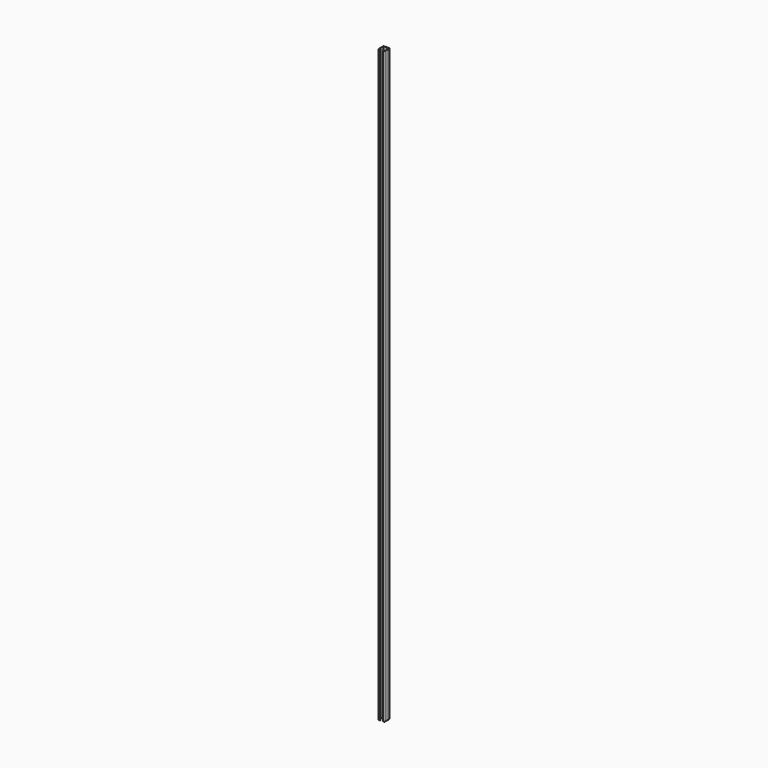
from build123d import *

# Parameters (mm, degrees)
F1_DEPTH    = 450
F2_T1_DEPTH = 452.5
F2_T3_DEPTH = 7.2
F3_R        = 0.5
F4_DEPTH    = 25


# Not quite as in the source:
# - a fillet or chamfer that OpenCascade refuses, or shapes differently, is made with other operations: its cross-section is extruded or revolved along the edge and cut away or added


with BuildPart() as f1:
    # F0 (on Top) → F1 (new body)
    with BuildSketch(Plane.XY):
        Polygon((-3.0933290763, 0), (-1.5933290763, 0), (-1.5933290763, 0.3), (-2.7933290763, 0.3), (-2.7933290763, 4.4), (1.6066709237, 4.4), (1.6066709237, 0.3), (0.4066709237, 0.3), (0.4066709237, 0), (1.9066709237, 0), (1.9066709237, 4.7), (-3.0933290763, 4.7), align=None)
    extrude(amount=F1_DEPTH)

    # F2: fillet of radius 0.5 on 8 edges, made by hand

    # F2_s2 → F2_t1 (cut)
    with BuildSketch(Plane.XY.offset(-1.25)):
        with BuildLine():
            ThreePointArc((-3.0933290763, 4.2), (-2.9468824669, 4.5535533906), (-2.5933290763, 4.7))
            Line((-2.5933290763, 4.7), (-3.0933290763, 4.7))
            Line((-3.0933290763, 4.7), (-3.0933290763, 4.2))
        make_face()
        with BuildLine():
            ThreePointArc((-3.0933290763, 0.5), (-2.9468824669, 0.1464466094), (-2.5933290763, 0))
            Line((-2.5933290763, 0), (-3.0933290763, 0))
            Line((-3.0933290763, 0), (-3.0933290763, 0.5))
        make_face()
        with BuildLine():
            ThreePointArc((1.4066709237, 0), (1.7602243143, 0.1464466094), (1.9066709237, 0.5))
            Line((1.9066709237, 0.5), (1.9066709237, 0))
            Line((1.9066709237, 0), (1.4066709237, 0))
        make_face()
        with BuildLine():
            ThreePointArc((1.9066709237, 4.2), (1.7602243143, 4.5535533906), (1.4066709237, 4.7))
            Line((1.4066709237, 4.7), (1.9066709237, 4.7))
            Line((1.9066709237, 4.7), (1.9066709237, 4.2))
        make_face()
    extrude(amount=F2_T1_DEPTH, mode=Mode.SUBTRACT)

    # F2_s4 → F2_t3 (cut)
    with BuildSketch(Plane.XZ.offset(-5.95)):
        with BuildLine():
            ThreePointArc((-3.0933290763, 0.5), (-2.9468824669, 0.1464466094), (-2.5933290763, 0))
            Line((-2.5933290763, 0), (-3.0933290763, 0))
            Line((-3.0933290763, 0), (-3.0933290763, 0.5))
        make_face()
        with BuildLine():
            ThreePointArc((-3.0933290763, 449.5), (-2.9468824669, 449.8535533906), (-2.5933290763, 450))
            Line((-2.5933290763, 450), (-3.0933290763, 450))
            Line((-3.0933290763, 450), (-3.0933290763, 449.5))
        make_face()
        with BuildLine():
            ThreePointArc((1.9066709237, 0.5), (1.7602243143, 0.1464466094), (1.4066709237, 0))
            Line((1.4066709237, 0), (1.9066709237, 0))
            Line((1.9066709237, 0), (1.9066709237, 0.5))
        make_face()
        with BuildLine():
            ThreePointArc((1.9066709237, 449.5), (1.7602243143, 449.8535533906), (1.4066709237, 450))
            Line((1.4066709237, 450), (1.9066709237, 450))
            Line((1.9066709237, 450), (1.9066709237, 449.5))
        make_face()
    extrude(amount=F2_T3_DEPTH, mode=Mode.SUBTRACT)

    # F3 (on face) → F4 (cut)
    with BuildSketch(Plane(origin=(0, 4.7, 0), x_dir=(-1, 0, 0), z_dir=(0, 1, 0))):
        with Locations((0.5933290763, 400)):
            Circle(F3_R)
        with Locations((0.5933290763, 391)):
            Circle(F3_R)
        with Locations((0.5933290763, 50)):
            Circle(F3_R)
        with Locations((0.5933290763, 59)):
            Circle(F3_R)
    extrude(amount=-F4_DEPTH, mode=Mode.SUBTRACT)


solid = f1.part
